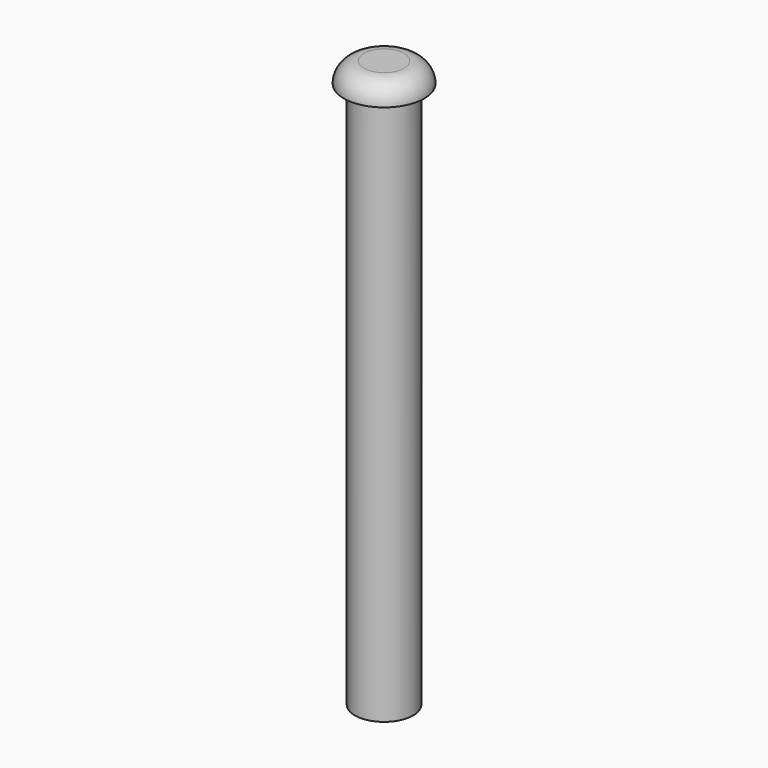
from build123d import *

# Parameters (mm, degrees)
F0_R     = 3.683
F1_DEPTH = 69.088
F2_R     = 5.08
F3_DEPTH = 2.54
F4_R     = 2.53999
F5_R     = 2.54
F6_DEPTH = 12.7


# Not quite as in the source:
# - a fillet or chamfer is up to 0.001 mm smaller than in the source, because OpenCascade refuses the exact size


with BuildPart() as f1:
    # F0 (on Top) → F1 (new body)
    with BuildSketch(Plane.XY):
        Circle(F0_R)
    extrude(amount=F1_DEPTH)

    # F2 (on face) → F3 (join)
    with BuildSketch(Plane.XY.offset(69.088)):
        Circle(F2_R)
    extrude(amount=F3_DEPTH)

    # F4 (radius 2.54 in the source; OpenCascade refuses exactly that, so slightly less here)
    f4_edges = [f1.edges().sort_by_distance(p)[0] for p in [
        (-5.08, 0, 71.628),
    ]]
    fillet(f4_edges, radius=F4_R)

    # F5 (on face) → F6 (cut)
    with BuildSketch(Plane(origin=(0, 0, 0), x_dir=(1, 0, 0), z_dir=(0, 0, -1))):
        Circle(F5_R)
    extrude(amount=-F6_DEPTH, mode=Mode.SUBTRACT)


solid = f1.part
